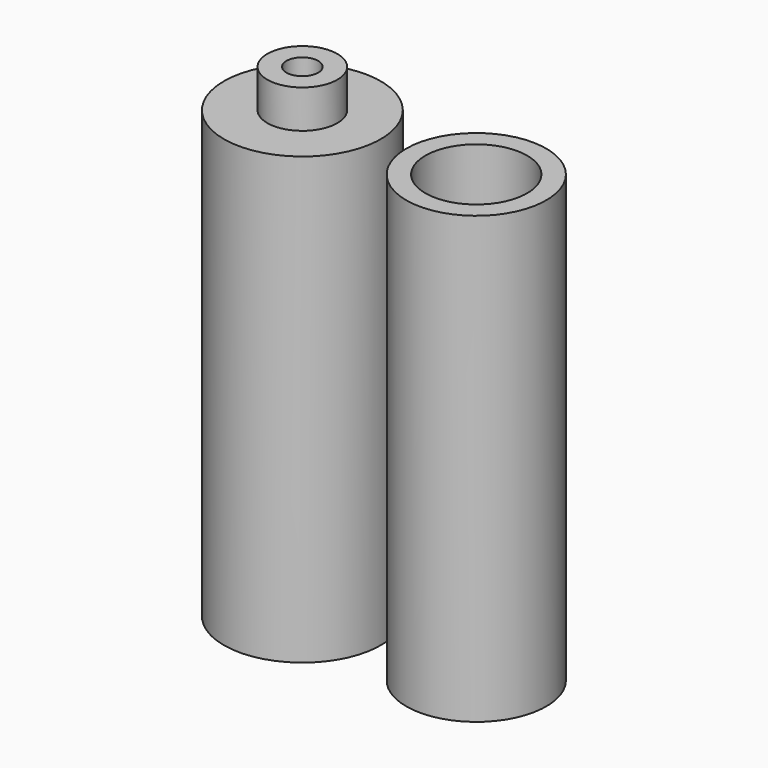
from build123d import *

# Parameters (mm, degrees)
F0_W   = 3
F0_H   = 6
F0_H_2 = 4


# Not quite as in the source:
# - a feature of the source that left no trace in its solid (it failed there, or was rolled back) is left out


with BuildPart() as f1:
    # F0 (on Front) → F1 (revolve)
    with BuildSketch(Plane.XZ):
        with BuildLine():
            Line((-8.325, -22.0375), (-8.325, 25.8375))
            ThreePointArc((-8.325, 25.8375), (-6.7126047478, 30.7615798633), (-2.5, 33.7782572057))
            Line((-2.5, 33.7782572057), (-2.5, 37.1625))
            Line((-2.5, 37.1625), (-5.5, 37.1625))
            Line((-5.5, 37.1625), (-12.325, 37.1625))
            Line((-12.325, 37.1625), (-12.325, -32.8375))
            Line((-12.325, -32.8375), (0, -32.8375))
            Line((0, -32.8375), (0, -26.8375))
            Line((0, -26.8375), (0, -25.8375))
            Line((0, -25.8375), (-8.325, -25.8375))
            Line((-8.325, -25.8375), (-10.325, -25.8375))
            Line((-10.325, -25.8375), (-10.325, -22.0375))
            Line((-10.325, -22.0375), (-8.325, -22.0375))
        make_face()
        with Locations((-4, 40.1625)):
            Rectangle(F0_W, F0_H)
    revolve(axis=Axis((0, 0, -29.3375), (0, 0, -1)))


with BuildPart() as f4:
    # F0 (on Front) → F4 (revolve)
    with BuildSketch(Plane.XZ):
        Polygon((19.325, 33.1625), (16.325, 33.1625), (16.325, -32.8375), (27.325, -32.8375), (27.325, -29.8375), (19.325, -29.8375), align=None)
        with Locations((17.825, 35.1625)):
            Rectangle(F0_W, F0_H_2)
    revolve(axis=Axis((27.325, 0, -31.3375), (0, 0, 1)))


solid = Compound([f1.part, f4.part])
